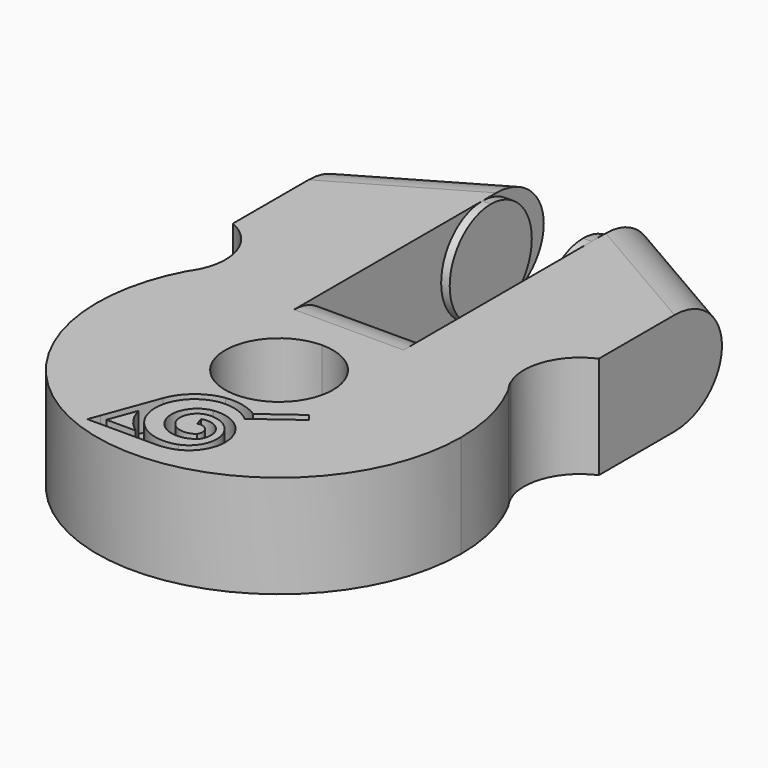
from build123d import *

# Parameters (mm, degrees)
F1_DEPTH  = 6
F3_DEPTH  = 0.5
F5_DEPTH  = 0.5
F6_R      = 2.99999
F7_R      = 2.99999
F9_DEPTH  = 1.5
F11_DEPTH = 1.5


# Not quite as in the source:
# - a fillet or chamfer is up to 0.001 mm smaller than in the source, because OpenCascade refuses the exact size


with BuildPart() as f1:
    # F0 (on Top) → F1 (new body)
    with BuildSketch(Plane.XY):
        with BuildLine():
            ThreePointArc((-21.257927263, 3.0925971456), (-19.5135237331, 1.2849088277), (-19.5663380414, -1.2266427602))
            ThreePointArc((-19.5663380414, -1.2266427602), (-17.0596555887, 1.5276447909), (-13.757927263, 3.2504758611))
            Line((-13.757927263, 3.2504758611), (-13.757927263, 16.4425971456))
            Line((-13.757927263, 16.4425971456), (-21.257927263, 12.0925971456))
            Line((-21.257927263, 12.0925971456), (-21.257927263, 3.0925971456))
        make_face()
        with BuildLine():
            ThreePointArc((-19.937029438, -1.8621137259), (-13.1593751133, -17.2347921219), (0.092072737, -6.9074028544))
            ThreePointArc((0.092072737, -6.9074028544), (-0.2305379955, -4.3059550041), (-1.178825088, -1.8621137259))
            ThreePointArc((-1.178825088, -1.8621137259), (-1.3821012217, -1.5548376637), (-1.5495164847, -1.2266427602))
            ThreePointArc((-1.5495164847, -1.2266427602), (-4.0561989374, 1.5276447909), (-7.357927263, 3.2504758611))
            Line((-7.357927263, 3.2504758611), (-7.357927263, 1.1925971456))
            Line((-7.357927263, 1.1925971456), (-10.557927263, 1.1925971456))
            Line((-10.557927263, 1.1925971456), (-13.757927263, 1.1925971456))
            Line((-13.757927263, 1.1925971456), (-13.757927263, 3.2504758611))
            ThreePointArc((-13.757927263, 3.2504758611), (-17.0596555887, 1.5276447909), (-19.5663380414, -1.2266427602))
            ThreePointArc((-19.5663380414, -1.2266427602), (-19.7337533043, -1.5548376637), (-19.937029438, -1.8621137259))
        make_face()
        with BuildLine():
            ThreePointArc((-7.407927263, -6.9074028544), (-12.7853136237, -9.1347892152), (-10.557927263, -3.7574028544))
            ThreePointArc((-10.557927263, -3.7574028544), (-8.3305409023, -4.6800164937), (-7.407927263, -6.9074028544))
        make_face(mode=Mode.SUBTRACT)
        with BuildLine():
            ThreePointArc((-7.357927263, 3.2504758611), (-4.0561989374, 1.5276447909), (-1.5495164847, -1.2266427602))
            ThreePointArc((-1.5495164847, -1.2266427602), (-1.6023307929, 1.2849088277), (0.142072737, 3.0925971456))
            Line((0.142072737, 3.0925971456), (0.142072737, 12.0925971456))
            Line((0.142072737, 12.0925971456), (-7.357927263, 16.4425971456))
            Line((-7.357927263, 16.4425971456), (-7.357927263, 3.2504758611))
        make_face()
    extrude(amount=F1_DEPTH)

    # F2 (on face) → F3 (join)
    with BuildSketch(Plane.YZ.offset(-13.757927263)):
        with BuildLine():
            ThreePointArc((11.9425971456, 0), (14.0639174891, 0.8786796564), (14.9425971456, 3))
            ThreePointArc((14.9425971456, 3), (14.0639174891, 5.1213203436), (11.9425971456, 6))
            ThreePointArc((11.9425971456, 6), (8.9425971456, 3), (11.9425971456, 0))
        make_face()
    extrude(amount=F3_DEPTH)

    # F4 (on face) → F5 (join)
    with BuildSketch(Plane(origin=(-7.357927263, 0, 0), x_dir=(0, -1, 0), z_dir=(-1, 0, 0))):
        with BuildLine():
            ThreePointArc((-11.9425971456, 0), (-9.821276802, 0.8786796564), (-8.9425971456, 3))
            ThreePointArc((-8.9425971456, 3), (-9.821276802, 5.1213203436), (-11.9425971456, 6))
            ThreePointArc((-11.9425971456, 6), (-14.9425971456, 3), (-11.9425971456, 0))
        make_face()
    extrude(amount=F5_DEPTH)

    # F6 (radius 3 in the source; OpenCascade refuses exactly that, so slightly less here)
    f6_edges = [f1.edges().sort_by_distance(p)[0] for p in [
        (-10.557927, 1.192597, 0),
        (-10.557927, 1.192597, 6),
    ]]
    fillet(f6_edges, radius=F6_R)

    # F7 (radius 3 in the source; OpenCascade refuses exactly that, so slightly less here)
    f7_edges = [f1.edges().sort_by_distance(p)[0] for p in [
        (-3.607927, 14.267597, 6),
        (-3.607927, 14.267597, 0),
        (-17.507927, 14.267597, 6),
        (-17.507927, 14.267597, 0),
    ]]
    fillet(f7_edges, radius=F7_R)

    # F8 (on face) → F9 (cut)
    with BuildSketch(Plane.XY.offset(6)):
        with BuildLine():
            ThreePointArc((-10.3315528874, -12.4037176265), (-8.5586184667, -13.6203290978), (-9.5390766145, -15.534001419))
            ThreePointArc((-9.5390766145, -15.534001419), (-12.5657731947, -13.9373786235), (-10.6819972396, -11.0805473911))
            ThreePointArc((-10.6819972396, -11.0805473911), (-9.6634977684, -11.1643464321), (-8.7690087855, -11.6585659294))
            Line((-8.7690087855, -11.6585659294), (-6.4111007419, -9.9150485592))
            Line((-6.4111007419, -9.9150485592), (-6.7083751907, -9.5130188313))
            Line((-6.7083751907, -9.5130188313), (-8.7669816313, -11.0352224208))
            ThreePointArc((-8.7669816313, -11.0352224208), (-9.7165335049, -10.6334325304), (-10.7464416358, -10.5847178642))
            ThreePointArc((-10.7464416358, -10.5847178642), (-10.7524542145, -10.5858192208), (-10.7585352096, -10.5864401769))
            ThreePointArc((-10.7585352096, -10.5864401769), (-12.1066928754, -11.1876295757), (-12.9640803834, -12.3892303605))
            Line((-12.9640803834, -12.3892303605), (-14.113424494, -15.4995148073))
            Line((-14.113424494, -15.4995148073), (-14.3623176984, -16.1730543119))
            Line((-14.3623176984, -16.1730543119), (-13.6445064842, -16.1730543119))
            Line((-13.6445064842, -16.1730543119), (-10.3284124834, -16.1730543119))
            ThreePointArc((-10.3284124834, -16.1730543119), (-9.8409208438, -16.1304430443), (-9.3682147094, -16.0039016311))
            ThreePointArc((-9.3682147094, -16.0039016311), (-9.361792524, -16.0016997739), (-9.355524465, -15.9990913118))
            ThreePointArc((-9.355524465, -15.9990913118), (-8.073910256, -13.497618257), (-10.3914165669, -11.9073142221))
            ThreePointArc((-10.3914165669, -11.9073142221), (-10.4058889802, -11.9084903608), (-10.4200689017, -11.9116150811))
            ThreePointArc((-10.4200689017, -11.9116150811), (-11.528535351, -14.0033516217), (-9.233119707, -14.5822528616))
            ThreePointArc((-9.233119707, -14.5822528616), (-9.1701495178, -14.5297943991), (-9.1224097378, -14.46317572))
            ThreePointArc((-9.1224097378, -14.46317572), (-9.1661029488, -13.263231915), (-10.3166224177, -12.9196053972))
            Line((-10.3166224177, -12.9196053972), (-10.1537286636, -13.392326906))
            ThreePointArc((-10.1537286636, -13.392326906), (-9.561565173, -13.5691888225), (-9.5390766145, -14.1867906375))
            ThreePointArc((-9.5390766145, -14.1867906375), (-11.0716295176, -13.8002825215), (-10.3315528874, -12.4037176265))
        make_face()
        with BuildLine():
            ThreePointArc((-13.0496571933, -14.0633096924), (-12.6340614687, -14.9692167321), (-11.9283702953, -15.6730543119))
            Line((-11.9283702953, -15.6730543119), (-13.6445064842, -15.6730543119))
            Line((-13.6445064842, -15.6730543119), (-13.0496571933, -14.0633096924))
        make_face(mode=Mode.SUBTRACT)
    extrude(amount=-F9_DEPTH, mode=Mode.SUBTRACT)

    # F10 (on face) → F11 (cut)
    with BuildSketch(Plane(origin=(0, 0, 0), x_dir=(1, 0, 0), z_dir=(0, 0, -1))):
        with BuildLine():
            Line((-6.4111007419, 9.9150485592), (-8.7690087855, 11.6585659294))
            ThreePointArc((-8.7690087855, 11.6585659294), (-9.6634977684, 11.1643464321), (-10.6819972396, 11.0805473911))
            ThreePointArc((-10.6819972396, 11.0805473911), (-12.5657731947, 13.9373786235), (-9.5390766145, 15.534001419))
            ThreePointArc((-9.5390766145, 15.534001419), (-8.5586184667, 13.6203290978), (-10.3315528874, 12.4037176265))
            ThreePointArc((-10.3315528874, 12.4037176265), (-11.0716295176, 13.8002825215), (-9.5390766145, 14.1867906375))
            ThreePointArc((-9.5390766145, 14.1867906375), (-9.561565173, 13.5691888225), (-10.1537286636, 13.392326906))
            Line((-10.1537286636, 13.392326906), (-10.3166224177, 12.9196053972))
            ThreePointArc((-10.3166224177, 12.9196053972), (-9.1661029488, 13.263231915), (-9.1224097378, 14.46317572))
            ThreePointArc((-9.1224097378, 14.46317572), (-9.1701495178, 14.5297943991), (-9.233119707, 14.5822528616))
            ThreePointArc((-9.233119707, 14.5822528616), (-11.528535351, 14.0033516217), (-10.4200689017, 11.9116150811))
            ThreePointArc((-10.4200689017, 11.9116150811), (-10.4058889802, 11.9084903608), (-10.3914165669, 11.9073142221))
            ThreePointArc((-10.3914165669, 11.9073142221), (-8.073910256, 13.497618257), (-9.355524465, 15.9990913118))
            ThreePointArc((-9.355524465, 15.9990913118), (-9.361792524, 16.0016997739), (-9.3682147094, 16.0039016311))
            ThreePointArc((-9.3682147094, 16.0039016311), (-9.8409208438, 16.1304430443), (-10.3284124834, 16.1730543119))
            Line((-10.3284124834, 16.1730543119), (-14.3623176984, 16.1730543119))
            Line((-14.3623176984, 16.1730543119), (-12.9640803834, 12.3892303605))
            ThreePointArc((-12.9640803834, 12.3892303605), (-12.1066928754, 11.1876295757), (-10.7585352096, 10.5864401769))
            ThreePointArc((-10.7585352096, 10.5864401769), (-10.7524542145, 10.5858192208), (-10.7464416358, 10.5847178642))
            ThreePointArc((-10.7464416358, 10.5847178642), (-9.7165335049, 10.6334325304), (-8.7669816313, 11.0352224208))
            Line((-8.7669816313, 11.0352224208), (-6.7083751907, 9.5130188313))
            Line((-6.7083751907, 9.5130188313), (-6.4111007419, 9.9150485592))
        make_face()
        with BuildLine():
            ThreePointArc((-11.9283702953, 15.6730543119), (-12.6340614687, 14.9692167321), (-13.0496571933, 14.0633096924))
            Line((-13.0496571933, 14.0633096924), (-13.6445064842, 15.6730543119))
            Line((-13.6445064842, 15.6730543119), (-11.9283702953, 15.6730543119))
        make_face(mode=Mode.SUBTRACT)
    extrude(amount=-F11_DEPTH, mode=Mode.SUBTRACT)


solid = f1.part
